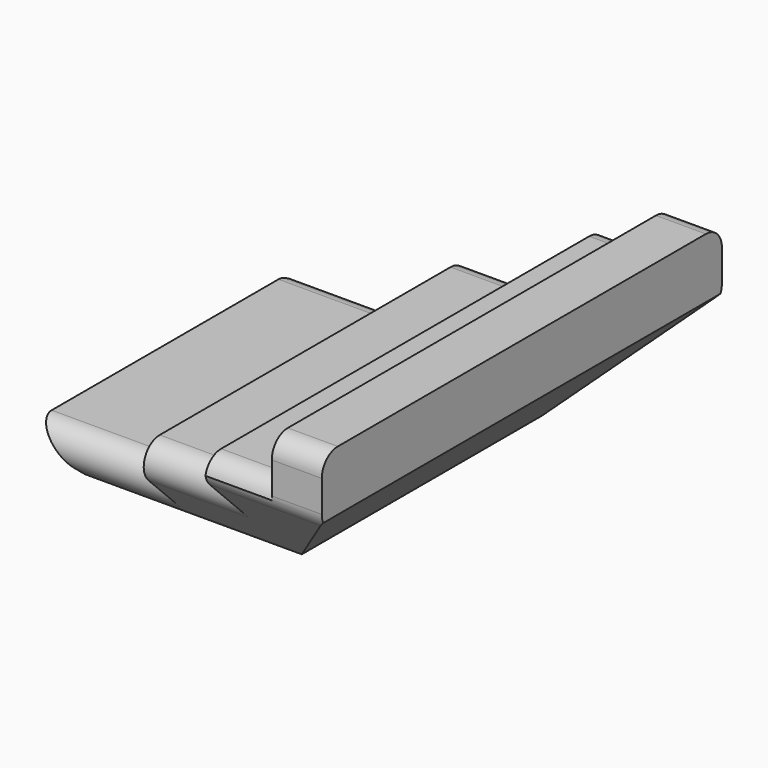
from build123d import *

# Parameters (mm, degrees)
F2_DEPTH    = 12.5
F3_T1_DEPTH = 46.550163213
F3_T3_DEPTH = 50.7168298797
F4_R        = 1
F4_R_2      = 0.99999


# Not quite as in the source:
# - a fillet or chamfer that OpenCascade refuses, or shapes differently, is made with other operations: its cross-section is extruded or revolved along the edge and cut away or added
# - a fillet or chamfer is up to 0.001 mm smaller than in the source, because OpenCascade refuses the exact size


with BuildPart() as f2:
    # F1 (on Front) → F2 (new body, symmetric)
    with BuildSketch(Plane.XZ):
        Polygon((0, 2), (0, 0), (20.8333333333, 0), (20.8333333333, 8), (18.3333333333, 8), (18.3333333333, 6), (15, 6), (15, 4), (10, 4), (10, 2), align=None)
    extrude(amount=F2_DEPTH, both=True)

    # F3: chamfer of 5 on 4 edges, made by hand

    # F3_s2 → F3_t1 (cut)
    with BuildSketch(Plane.YZ.offset(-12.8584149398)):
        Polygon((-12.5, 5), (-7.5, 0), (-12.5, 0), align=None)
        Polygon((7.5, 0), (12.5, 5), (12.5, 0), align=None)
    extrude(amount=F3_T1_DEPTH, mode=Mode.SUBTRACT)

    # F3_s4 → F3_t3 (cut)
    with BuildSketch(Plane.XZ.offset(-25.3584149398)):
        Polygon((0, 5), (5, 0), (0, 0), align=None)
        Polygon((20.8333333333, 5), (15.8333333333, 0), (20.8333333333, 0), align=None)
    extrude(amount=F3_T3_DEPTH, mode=Mode.SUBTRACT)

    # F4 (call 1 of 10: OpenCascade refuses the feature's edges together)
    f4_edges = [f2.edges().sort_by_distance(p)[0] for p in [
        (6.5, -9.5, 2),
    ]]
    fillet(f4_edges, radius=F4_R)

    # F4#2 (call 2 of 10)
    f4_2_edges = [f2.edges().sort_by_distance(p)[0] for p in [
        (12.5, -11.5, 4),
    ]]
    fillet(f4_2_edges, radius=F4_R)

    # F4#3 (call 3 of 10) (radius 1 in the source; OpenCascade refuses exactly that, so slightly less here)
    f4_3_edges = [f2.edges().sort_by_distance(p)[0] for p in [
        (16.666667, -12.5, 6),
    ]]
    fillet(f4_3_edges, radius=F4_R_2)

    # F4#4 (call 4 of 10)
    f4_4_edges = [f2.edges().sort_by_distance(p)[0] for p in [
        (19.583333, -12.5, 8),
    ]]
    fillet(f4_4_edges, radius=F4_R)

    # F4#5 (call 5 of 10)
    f4_5_edges = [f2.edges().sort_by_distance(p)[0] for p in [
        (19.583333, 12.5, 8),
    ]]
    fillet(f4_5_edges, radius=F4_R)

    # F4#6 (call 6 of 10) (radius 1 in the source; OpenCascade refuses exactly that, so slightly less here)
    f4_6_edges = [f2.edges().sort_by_distance(p)[0] for p in [
        (16.666667, 12.5, 6),
    ]]
    fillet(f4_6_edges, radius=F4_R_2)

    # F4#7 (call 7 of 10)
    f4_7_edges = [f2.edges().sort_by_distance(p)[0] for p in [
        (12.5, 11.5, 4),
    ]]
    fillet(f4_7_edges, radius=F4_R)

    # F4#8 (call 8 of 10)
    f4_8_edges = [f2.edges().sort_by_distance(p)[0] for p in [
        (6.5, 9.5, 2),
    ]]
    fillet(f4_8_edges, radius=F4_R)

    # F4#9 (call 9 of 10)
    f4_9_edges = [f2.edges().sort_by_distance(p)[0] for p in [
        (17.916667, -12.5, 5),
    ]]
    fillet(f4_9_edges, radius=F4_R)

    # F4#10 (call 10 of 10)
    f4_10_edges = [f2.edges().sort_by_distance(p)[0] for p in [
        (17.916667, 12.5, 5),
    ]]
    fillet(f4_10_edges, radius=F4_R)


solid = f2.part
